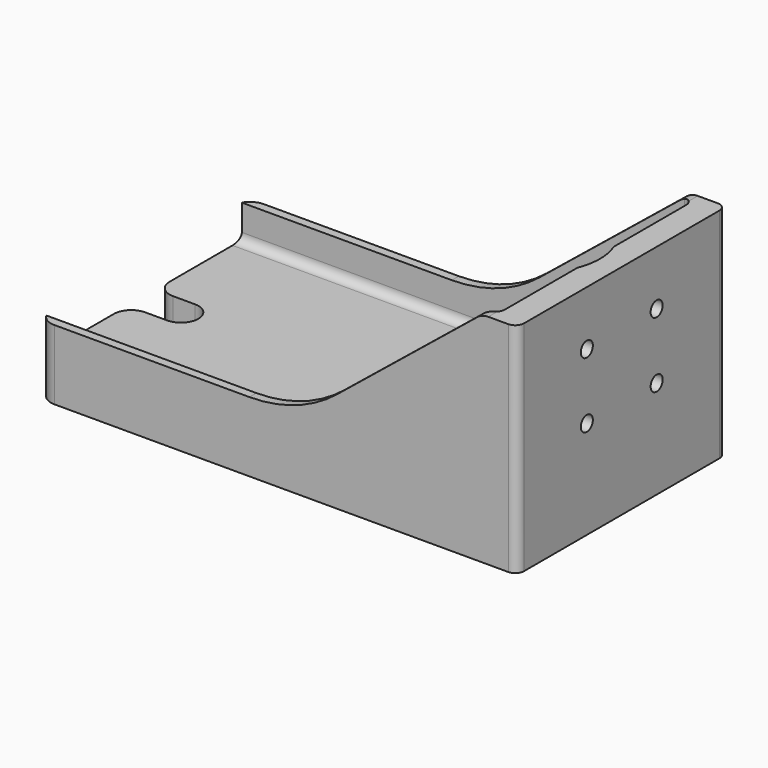
from build123d import *

# Parameters (mm, degrees)
F0_W      = 110
F0_H      = 60
F1_DEPTH  = 8
F3_DEPTH  = 2
F5_DEPTH  = 2
F6_W      = 6
F6_H      = 56
F7_DEPTH  = 42
F8_W      = 13
F8_H      = 8
F9_DEPTH  = 8
F10_R     = 3.99999
F11_R     = 2
F12_R     = 1.725
F13_DEPTH = 6
F12_R_2   = 3.5
F14_DEPTH = 3
F17_R     = 5.5
F18_DEPTH = 8
F19_R     = 1.725
F20_DEPTH = 8
F19_R_2   = 14
F21_DEPTH = 55
F22_R     = 32


# Not quite as in the source:
# - a fillet or chamfer is up to 0.001 mm smaller than in the source, because OpenCascade refuses the exact size


with BuildPart() as f1:
    # F0 (on Top) → F1 (new body)
    with BuildSketch(Plane.XY):
        with Locations((55, 30)):
            Rectangle(F0_W, F0_H)
    extrude(amount=F1_DEPTH)

    # F2 (on face) → F3 (join)
    with BuildSketch(Plane.XZ):
        Polygon((0, 8), (110, 8), (110, 50), (102, 50), (60, 16), (0, 16), align=None)
    extrude(amount=-F3_DEPTH)

    # F4 (on face) → F5 (join)
    with BuildSketch(Plane(origin=(0, 60, 0), x_dir=(-1, 0, 0), z_dir=(0, 1, 0))):
        Polygon((-110, 50), (-110, 8), (0, 8), (0, 16), (-60, 16), (-102, 50), align=None)
    extrude(amount=-F5_DEPTH)

    # F6 (on face) → F7 (join)
    with BuildSketch(Plane.XY.offset(8)):
        with Locations((107, 30)):
            Rectangle(F6_W, F6_H)
    extrude(amount=F7_DEPTH)

    # F8 (on face) → F9 (cut)
    with BuildSketch(Plane.XY.offset(8)):
        with Locations((6.5, 30)):
            Rectangle(F8_W, F8_H)
    extrude(amount=-F9_DEPTH, mode=Mode.SUBTRACT)

    # F10 (radius 4 in the source; OpenCascade refuses exactly that, so slightly less here)
    f10_edges = [f1.edges().sort_by_distance(p)[0] for p in [
        (102, 59, 50),
        (102, 1, 50),
        (0, 60, 8),
        (0, 34, 4),
        (0, 26, 4),
        (13, 26, 4),
        (13, 34, 4),
        (0, 0, 8),
    ]]
    fillet(f10_edges, radius=F10_R)

    # F11
    f11_edges = [f1.edges().sort_by_distance(p)[0] for p in [
        (52.267947, 58, 8),
        (52.267947, 2, 8),
        (110, 0, 25),
        (110, 60, 25),
        (104, 2, 29),
        (104, 58, 29),
        (104, 30, 8),
    ]]
    fillet(f11_edges, radius=F11_R)

    # F12 (on face) → F13 (cut)
    with BuildSketch(Plane.YZ.offset(110)):
        with Locations((20, 37.5)):
            Circle(F12_R)
        with Locations((40, 22.5)):
            Circle(F12_R)
        with Locations((20, 22.5)):
            Circle(F12_R)
        with Locations((40, 37.5)):
            Circle(F12_R)
    extrude(amount=-F13_DEPTH, mode=Mode.SUBTRACT)


with BuildPart() as f14:
    # F12 (on face) → F14 (new body)
    with BuildSketch(Plane.YZ.offset(110)):
        with Locations((20, 22.5)):
            Circle(F12_R_2)
        with Locations((20, 22.5)):
            Circle(F12_R, mode=Mode.SUBTRACT)
    extrude(amount=-F14_DEPTH)


with BuildPart() as f14b:
    # F12 (on face) → F14, piece 2 (new body)
    with BuildSketch(Plane.YZ.offset(110)):
        with Locations((40, 22.5)):
            Circle(F12_R_2)
        with Locations((40, 22.5)):
            Circle(F12_R, mode=Mode.SUBTRACT)
    extrude(amount=-F14_DEPTH)


with BuildPart() as f14c:
    # F12 (on face) → F14, piece 3 (new body)
    with BuildSketch(Plane.YZ.offset(110)):
        with Locations((40, 37.5)):
            Circle(F12_R_2)
        with Locations((40, 37.5)):
            Circle(F12_R, mode=Mode.SUBTRACT)
    extrude(amount=-F14_DEPTH)


with BuildPart() as f14d:
    # F12 (on face) → F14, piece 4 (new body)
    with BuildSketch(Plane.YZ.offset(110)):
        with Locations((20, 37.5)):
            Circle(F12_R_2)
        with Locations((20, 37.5)):
            Circle(F12_R, mode=Mode.SUBTRACT)
    extrude(amount=-F14_DEPTH)


with BuildPart() as f14d_1:
    # F15: moved
    add(f14d.part.moved(Location((-4, 0, 0))))


with BuildPart() as f14c_1:
    # F15: moved
    add(f14c.part.moved(Location((-4, 0, 0))))


with BuildPart() as f14b_1:
    # F15: moved
    add(f14b.part.moved(Location((-4, 0, 0))))


with BuildPart() as f14_1:
    # F15: moved
    add(f14.part.moved(Location((-4, 0, 0))))


with BuildPart() as f1_1:
    add(f1.part)

    # F16: cut F14d, F14c, F14b, F14
    add(f14d_1.part, mode=Mode.SUBTRACT)
    add(f14c_1.part, mode=Mode.SUBTRACT)
    add(f14b_1.part, mode=Mode.SUBTRACT)
    add(f14_1.part, mode=Mode.SUBTRACT)

    # F17 (on face) → F18 (cut)
    with BuildSketch(Plane(origin=(0, 0, 0), x_dir=(1, 0, 0), z_dir=(0, 0, -1))):
        with Locations((91, -30)):
            Circle(F17_R)
    extrude(amount=-F18_DEPTH, mode=Mode.SUBTRACT)

    # F19 (on face) → F20 (cut)
    with BuildSketch(Plane.XY.offset(8)):
        with Locations((91, 37.6)):
            Circle(F19_R)
        with Locations((91, 22.4)):
            Circle(F19_R)
    extrude(amount=-F20_DEPTH, mode=Mode.SUBTRACT)

    # F19 (on face) → F21 (cut)
    with BuildSketch(Plane.XY.offset(8)):
        with Locations((91, 30)):
            Circle(F19_R_2)
        with Locations((91, 22.4)):
            Circle(F19_R, mode=Mode.SUBTRACT)
        with Locations((83.4, 30)):
            Circle(F19_R, mode=Mode.SUBTRACT)
        with Locations((91, 37.6)):
            Circle(F19_R, mode=Mode.SUBTRACT)
        with Locations((98.6, 30)):
            Circle(F19_R, mode=Mode.SUBTRACT)
        with Locations((-18, 77.4)):
            Circle(F19_R)
        with Locations((-77.4, -18)):
            Circle(F19_R)
        with Locations((18, -77.4)):
            Circle(F19_R)
        with Locations((98.6, 30)):
            Circle(F19_R)
    extrude(amount=F21_DEPTH, mode=Mode.SUBTRACT)

    # F22
    f22_edges = [f1_1.edges().sort_by_distance(p)[0] for p in [
        (60, 59, 16),
        (60, 1, 16),
    ]]
    fillet(f22_edges, radius=F22_R)


solid = f1_1.part
